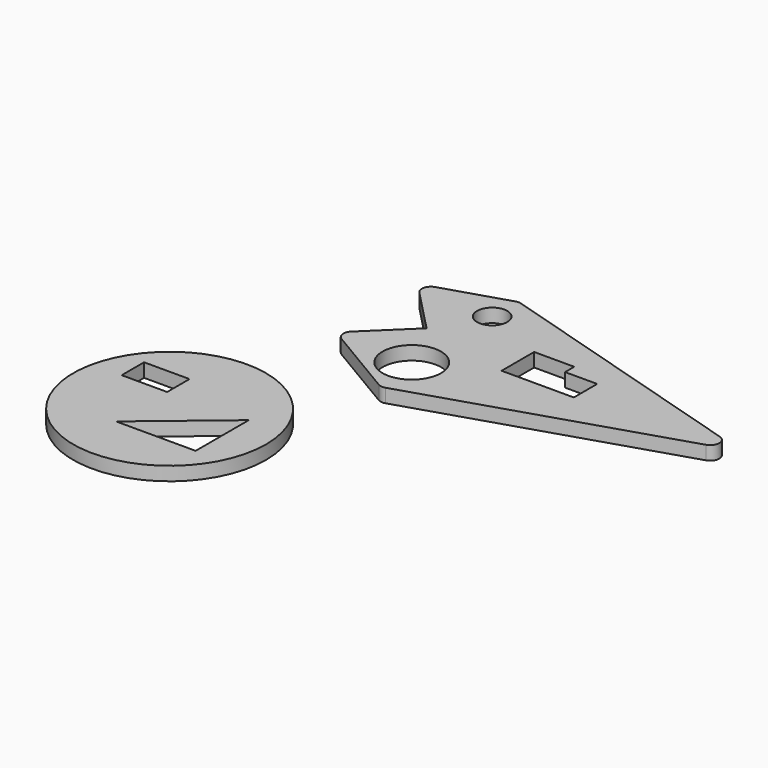
from build123d import *

# Parameters (mm, degrees)
F0_R     = 20.324324422
F0_R_2   = 10.4940599903
F1_DEPTH = 9.525
F2_R     = 67.0385979525
F2_W     = 31.5919071436
F2_H     = 19.4411873817
F3_DEPTH = 9.525


# Not quite as in the source:
# - a length typed as a fraction of an inch, garbled in the dataset ("3 / 203.2 mm" for 3/8 in), is restored


with BuildPart() as f1:
    # F0 (on Top) → F1 (new body)
    with BuildSketch(Plane.XY):
        with BuildLine():
            Line((128.5741976681, -0.0486427593), (-53.5251772372, 54.8306196901))
            ThreePointArc((-53.5251772372, 54.8306196901), (-55.3921510201, 55.100625175), (-57.2560646842, 54.8102462485))
            Line((-57.2560646842, 54.8102462485), (-101.960576079, 40.803295241))
            ThreePointArc((-101.960576079, 40.803295241), (-106.2154403374, 36.3114148976), (-104.6284180017, 30.3312628107))
            Line((-104.6284180017, 30.3312628107), (-75.319558382, 0))
            Line((-75.319558382, 0), (-104.8098202684, -28.4962070709))
            ThreePointArc((-104.8098202684, -28.4962070709), (-106.7047048987, -33.7970240568), (-103.6426431598, -38.5206906821))
            Line((-103.6426431598, -38.5206906821), (-54.2549128038, -67.8863703831))
            ThreePointArc((-54.2549128038, -67.8863703831), (-51.7372753813, -68.7364841392), (-49.0922061501, -68.4819250078))
            Line((-49.0922061501, -68.4819250078), (128.659276857, -12.1821500059))
            ThreePointArc((128.659276857, -12.1821500059), (133.0917430276, -6.0840179977), (128.5741976681, -0.0486427593))
        make_face()
        with Locations((-56.5892979503, -36.2649746239)):
            Circle(F0_R, mode=Mode.SUBTRACT)
        Polygon((-12.3540004715, -13.5495513678), (-12.3540004715, 14.7451004013), (15.5421346426, 14.7451004013), (15.5421346426, 6.7747756839), (37.8590412438, 6.7747756839), (37.8590412438, -13.5495513678), align=None, mode=Mode.SUBTRACT)
        with Locations((-56.1907812953, 33.0768451095)):
            Circle(F0_R_2, mode=Mode.SUBTRACT)
    extrude(amount=F1_DEPTH)


with BuildPart() as f3:
    # F2 (on Top) → F3 (new body)
    with BuildSketch(Plane.XY):
        with Locations((-125.1525729895, -160.9972268343)):
            Circle(F2_R)
        Polygon((-138.5183781385, -190.7665282488), (-83.2325294614, -144.5937305689), (-83.2325294614, -190.7665282488), align=None, mode=Mode.SUBTRACT)
        with Locations((-154.3143317103, -136.6957575083)):
            Rectangle(F2_W, F2_H, mode=Mode.SUBTRACT)
    extrude(amount=F3_DEPTH)


solid = Compound([f1.part, f3.part])
